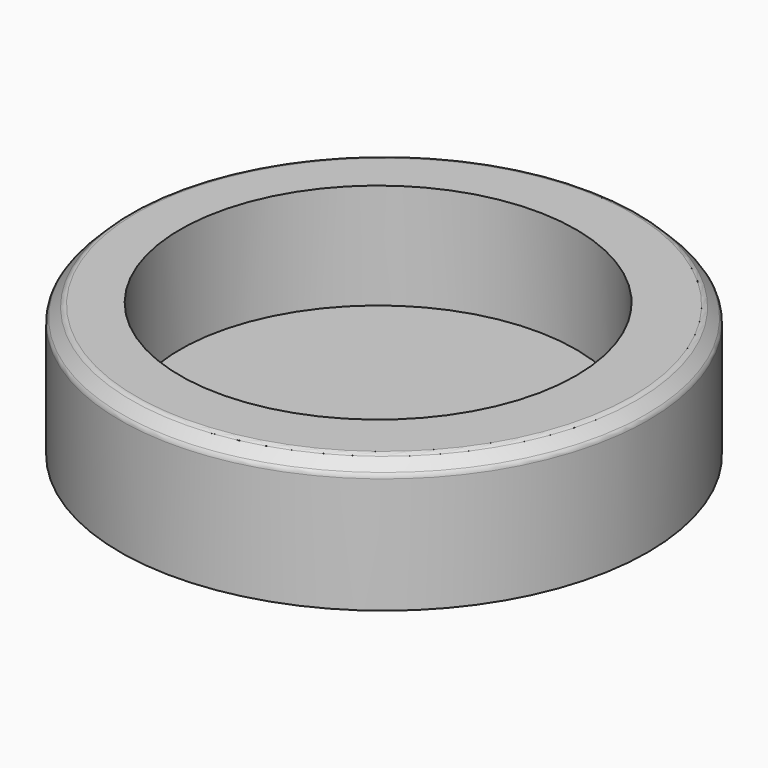
from build123d import *

# Parameters (mm, degrees)
F0_R     = 200
F1_DEPTH = 100
F2_R     = 150
F3_DEPTH = 80
F4_SIZE  = 10
F5_R     = 5
F6_R     = 5


with BuildPart() as f1:
    # F0 (on Top) → F1 (new body)
    with BuildSketch(Plane.XY):
        with Locations((4.4975979886, 0)):
            Circle(F0_R)
    extrude(amount=F1_DEPTH)

    # F2 (on face) → F3 (cut)
    with BuildSketch(Plane.XY.offset(100)):
        Circle(F2_R)
    extrude(amount=-F3_DEPTH, mode=Mode.SUBTRACT)

    # F4
    f4_edges = [f1.edges().sort_by_distance(p)[0] for p in [
        (-195.502402, 0, 100),
    ]]
    chamfer(f4_edges, length=F4_SIZE)

    # F5
    f5_edges = [f1.edges().sort_by_distance(p)[0] for p in [
        (-185.502402, 0, 100),
    ]]
    fillet(f5_edges, radius=F5_R)

    # F6
    f6_edges = [f1.edges().sort_by_distance(p)[0] for p in [
        (-195.502402, 0, 90),
    ]]
    fillet(f6_edges, radius=F6_R)


solid = f1.part
